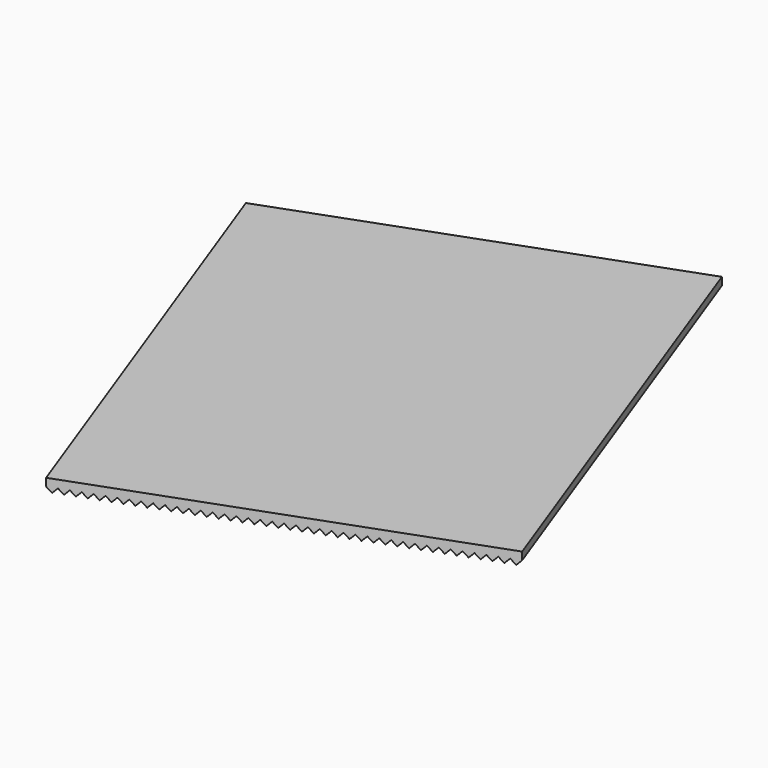
from build123d import *

# Parameters (mm, degrees)
F3_DEPTH = 254


# Not quite as in the source:
# - a feature of the source that left no trace in its solid (it failed there, or was rolled back) is left out


with BuildPart() as f3:
    # F2 (on face) → F3 (new body)
    with BuildSketch(Plane(origin=(0, 0, 0), x_dir=(-0.9390877837, -0.3436773698, 0), z_dir=(-0.3436773698, 0.9390877837, 0))):
        Polygon((-2.54, -2.54), (0, 0), (0, 4.0038675896), (-203.2, 4.0038675896), (-203.2, 0), (-200.66, -2.54), (-198.12, 0), (-195.58, -2.54), (-193.04, 0), (-190.5, -2.54), (-187.96, 0), (-185.42, -2.54), (-182.88, 0), (-180.34, -2.54), (-177.8, 0), (-175.26, -2.54), (-172.72, 0), (-170.18, -2.54), (-167.64, 0), (-165.1, -2.54), (-162.56, 0), (-160.02, -2.54), (-157.48, 0), (-154.94, -2.54), (-152.4, 0), (-149.86, -2.54), (-147.32, 0), (-144.78, -2.54), (-142.24, 0), (-139.7, -2.54), (-137.16, 0), (-134.62, -2.54), (-132.08, 0), (-129.54, -2.54), (-127, 0), (-124.46, -2.54), (-121.92, 0), (-119.38, -2.54), (-116.84, 0), (-114.3, -2.54), (-111.76, 0), (-109.22, -2.54), (-106.68, 0), (-104.14, -2.54), (-101.6, 0), (-99.06, -2.54), (-96.52, 0), (-93.98, -2.54), (-91.44, 0), (-88.9, -2.54), (-86.36, 0), (-83.82, -2.54), (-81.28, 0), (-78.74, -2.54), (-76.2, 0), (-73.66, -2.54), (-71.12, 0), (-68.58, -2.54), (-66.04, 0), (-63.5, -2.54), (-60.96, 0), (-58.42, -2.54), (-55.88, 0), (-53.34, -2.54), (-50.8, 0), (-48.26, -2.54), (-45.72, 0), (-43.18, -2.54), (-40.64, 0), (-38.1, -2.54), (-35.56, 0), (-33.02, -2.54), (-30.48, 0), (-27.94, -2.54), (-25.4, 0), (-22.86, -2.54), (-20.32, 0), (-17.78, -2.54), (-15.24, 0), (-12.7, -2.54), (-10.16, 0), (-7.62, -2.54), (-5.08, 0), align=None)
    extrude(amount=-F3_DEPTH)


solid = f3.part
